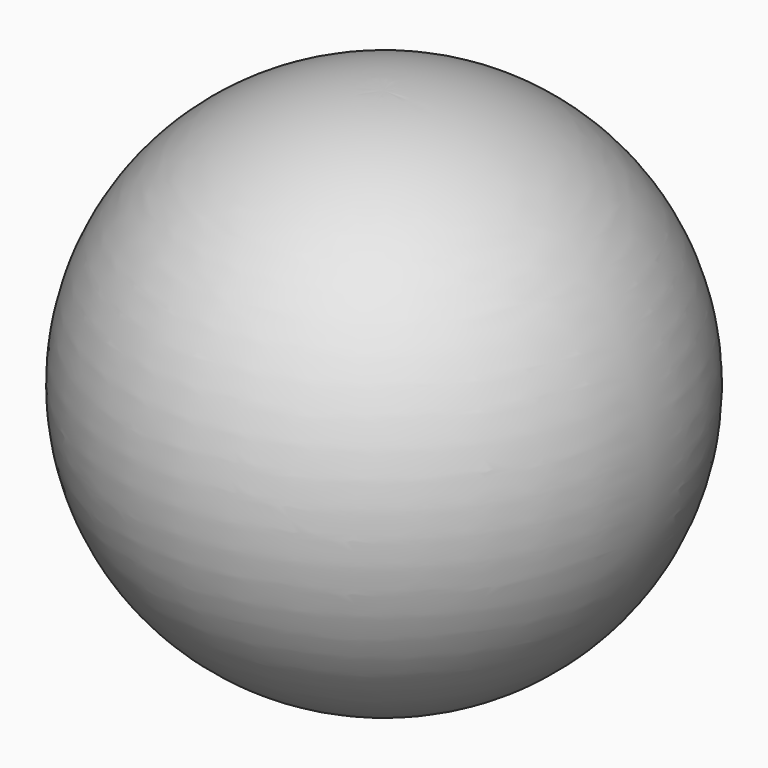
from build123d import *


# Not quite as in the source:
# - the program builds the solid bodies; features that only make, move or delete a surface that nothing else refers to are left out


with BuildPart() as f1:
    # F0 (on Front) → F1 (revolve)
    with BuildSketch(Plane.XZ):
        with BuildLine():
            ThreePointArc((0, -48.2004731894), (40.3211511153, -8.7510962039), (0, 30.6982807815))
            Line((0, 30.6982807815), (0, -48.2004731894))
        make_face()
    revolve(axis=Axis((0, 0, -8.7510962039), (0, 0, -1)))


solid = f1.part
